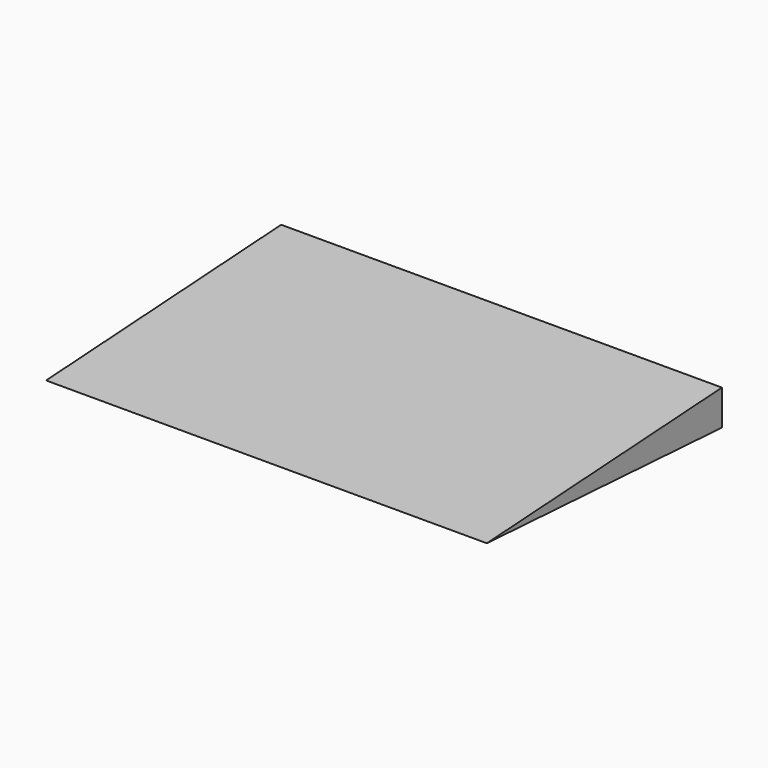
from build123d import *

# Parameters (mm, degrees)
F0_W     = 150
F0_H     = 100
F1_DEPTH = 12
F2_SIZE2 = 99.99999
F2_SIZE  = 5.99999


# Not quite as in the source:
# - a fillet or chamfer is up to 0.001 mm smaller than in the source, because OpenCascade refuses the exact size


with BuildPart() as f1:
    # F0 (on Top) → F1 (new body)
    with BuildSketch(Plane.XY):
        with Locations((-75, 50)):
            Rectangle(F0_W, F0_H)
    extrude(amount=F1_DEPTH)

    # F2 (size 6 and 100 in the source; OpenCascade refuses exactly that, so slightly less here)
    f2_edges = [f1.edges().sort_by_distance(p)[0] for p in [
        (-75, 0, 12),
        (-75, 0, 0),
    ]]
    f2_side = f1.faces().sort_by_distance((-75, 0, 6))[0]
    chamfer(f2_edges, length=F2_SIZE, length2=F2_SIZE2, reference=f2_side)


solid = f1.part
